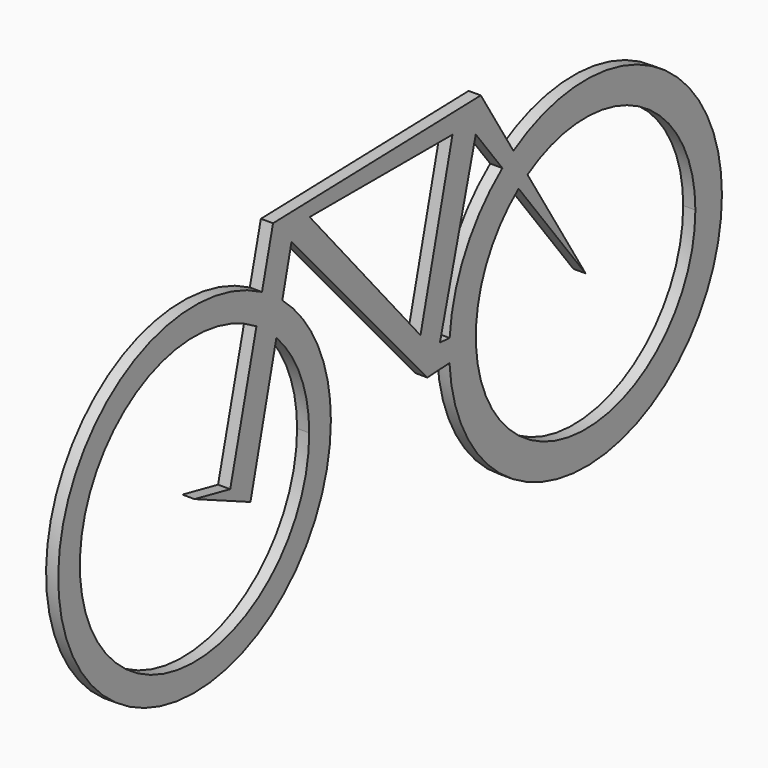
from build123d import *

# Parameters (mm, degrees)
F1_DEPTH = 12.7


with BuildPart() as f1:
    # F0 (on Right) → F1 (new body, symmetric)
    with BuildSketch(Plane.YZ):
        with BuildLine():
            ThreePointArc((-334.113415, 309.055447), (-817.405782, -178.754147), (-154.4, 0))
            ThreePointArc((-154.4, 0), (-187.635415, 150.108077), (-281.129104, 272.157074))
            Line((-281.129104, 272.157074), (-296.538995, 209.650203))
            ThreePointArc((-296.538995, 209.650203), (-233.065271, 113.251775), (-210.803061, 0))
            ThreePointArc((-210.803061, 0), (-772.516883, -143.539872), (-348.529702, 251.885195))
            Line((-348.529702, 251.885195), (-334.113415, 309.055447))
        make_face()
        with BuildLine():
            Line((224.114919, -16.312839), (154.977496, -20.257878))
            ThreePointArc((154.977496, -20.257878), (520.133054, -355.455597), (865.6, 0))
            ThreePointArc((865.6, 0), (682.514383, 310.950394), (321.785895, 301.706498))
            Line((321.785895, 301.706498), (358.438891, 242.951885))
            ThreePointArc((358.438891, 242.951885), (648.918766, 250.395616), (796.350115, 0))
            ThreePointArc((796.350115, 0), (518.159733, -286.233833), (224.114919, -16.312839))
        make_face()
        with BuildLine():
            Line((510, 0), (358.438891, 242.951885))
            ThreePointArc((358.438891, 242.951885), (346.633223, 235.175859), (335.225711, 226.826666))
            Line((335.225711, 226.826666), (510, 0))
        make_face()
        with BuildLine():
            ThreePointArc((155.322698, 25.600229), (154.410075, 2.676746), (154.977496, -20.257878))
            Line((154.977496, -20.257878), (224.114919, -16.312839))
            ThreePointArc((224.114919, -16.312839), (223.657998, 2.155474), (224.392896, 20.614816))
            Line((224.392896, 20.614816), (155.322698, 25.600229))
        make_face()
        with BuildLine():
            ThreePointArc((292.958924, 281.681614), (196.77501, 168.349236), (155.322698, 25.600229))
            Line((155.322698, 25.600229), (224.392896, 20.614816))
            ThreePointArc((224.392896, 20.614816), (257.772745, 135.564745), (335.225711, 226.826666))
            Line((335.225711, 226.826666), (292.958924, 281.681614))
        make_face()
        with BuildLine():
            Line((358.438891, 242.951885), (321.785895, 301.706498))
            ThreePointArc((321.785895, 301.706498), (307.125188, 292.049946), (292.958924, 281.681614))
            Line((292.958924, 281.681614), (335.225711, 226.826666))
            ThreePointArc((335.225711, 226.826666), (346.633223, 235.175859), (358.438891, 242.951885))
        make_face()
        with BuildLine():
            Line((-296.538995, 209.650203), (-281.129104, 272.157074))
            ThreePointArc((-281.129104, 272.157074), (-306.78207, 291.811297), (-334.113415, 309.055447))
            Line((-334.113415, 309.055447), (-348.529702, 251.885195))
            ThreePointArc((-348.529702, 251.885195), (-321.348684, 232.227236), (-296.538995, 209.650203))
        make_face()
        with BuildLine():
            ThreePointArc((-334.113415, 309.055447), (-306.78207, 291.811297), (-281.129104, 272.157074))
            Line((-281.129104, 272.157074), (-257.018694, 369.955702))
            Line((-257.018694, 369.955702), (-305.249922, 423.518568))
            Line((-305.249922, 423.518568), (-334.113415, 309.055447))
        make_face()
        with BuildLine():
            Line((-305.249922, 423.518568), (-257.018694, 369.955702))
            Line((-257.018694, 369.955702), (97.315804, -23.548102))
            Line((97.315804, -23.548102), (154.977496, -20.257878))
            ThreePointArc((154.977496, -20.257878), (154.410075, 2.676746), (155.322698, 25.600229))
            Line((155.322698, 25.600229), (130.044319, 27.424796))
            Line((130.044319, 27.424796), (223.514043, 371.809006))
            Line((223.514043, 371.809006), (292.958924, 281.681614))
            ThreePointArc((292.958924, 281.681614), (307.125188, 292.049946), (321.785895, 301.706498))
            Line((321.785895, 301.706498), (236.655169, 438.170731))
            Line((236.655169, 438.170731), (-305.249922, 423.518568))
        make_face()
        Polygon((79.300396, 61.445657), (-209.679782, 396.11885), (162.819028, 396.11885), align=None, mode=Mode.SUBTRACT)
        with BuildLine():
            Line((-364.150576, -64.601459), (-296.538995, 209.650203))
            ThreePointArc((-296.538995, 209.650203), (-321.348684, 232.227236), (-348.529702, 251.885195))
            Line((-348.529702, 251.885195), (-416.975014, -19.546399))
            Line((-416.975014, -19.546399), (-510, 0))
            Line((-510, 0), (-364.150576, -64.601459))
        make_face()
    extrude(amount=F1_DEPTH, both=True)


solid = f1.part
